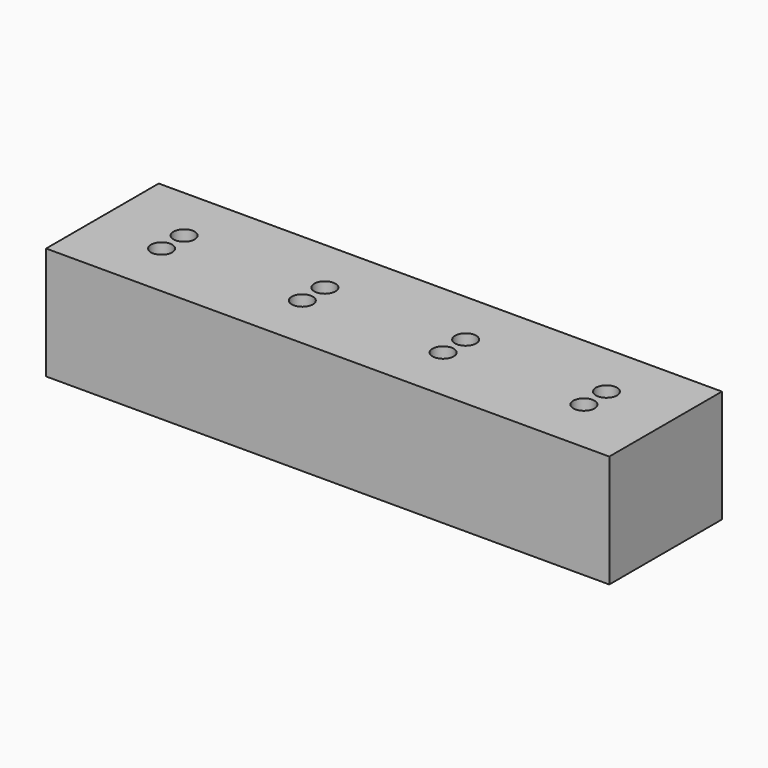
from build123d import *

# Parameters (mm, degrees)
F0_W     = 508
F0_H     = 127
F0_R     = 9.525
F1_DEPTH = 25.4
F3_DEPTH = 101.6


# Not quite as in the source:
# - a fillet or chamfer that OpenCascade refuses, or shapes differently, is made with other operations: its cross-section is extruded or revolved along the edge and cut away or added


with BuildPart() as f1:
    # F0 (on Top) → F1 (new body)
    with BuildSketch(Plane.XY):
        with Locations((254, 63.5)):
            Rectangle(F0_W, F0_H)
        with Locations((63.5, 50.8)):
            Circle(F0_R, mode=Mode.SUBTRACT)
        with Locations((190.5, 50.8)):
            Circle(F0_R, mode=Mode.SUBTRACT)
        with Locations((317.5, 50.8)):
            Circle(F0_R, mode=Mode.SUBTRACT)
        with Locations((444.5, 50.8)):
            Circle(F0_R, mode=Mode.SUBTRACT)
        with Locations((63.5, 76.2)):
            Circle(F0_R, mode=Mode.SUBTRACT)
        with Locations((190.5, 76.2)):
            Circle(F0_R, mode=Mode.SUBTRACT)
        with Locations((317.5, 76.2)):
            Circle(F0_R, mode=Mode.SUBTRACT)
        with Locations((444.5, 76.2)):
            Circle(F0_R, mode=Mode.SUBTRACT)
    extrude(amount=F1_DEPTH)

    # F2: fillet of radius 5.08 on 16 edges, made by hand

    # F2_s1 → F2_t2 (revolve, cut)
    with BuildSketch(Plane.XZ.offset(-76.2)):
        with BuildLine():
            ThreePointArc((200.025, 20.32), (201.5128975516, 23.9121024484), (205.105, 25.4))
            Line((205.105, 25.4), (200.025, 25.4))
            Line((200.025, 25.4), (200.025, 20.32))
        make_face()
    revolve(axis=Axis((190.5, 76.2, 25.4), (0, 0, 1)), mode=Mode.SUBTRACT)

    # F2_s3 → F2_t4 (revolve, cut)
    with BuildSketch(Plane.XZ.offset(-50.8)):
        with BuildLine():
            ThreePointArc((200.025, 20.32), (201.5128975516, 23.9121024484), (205.105, 25.4))
            Line((205.105, 25.4), (200.025, 25.4))
            Line((200.025, 25.4), (200.025, 20.32))
        make_face()
    revolve(axis=Axis((190.5, 50.8, 25.4), (0, 0, 1)), mode=Mode.SUBTRACT)

    # F2_s5 → F2_t6 (revolve, cut)
    with BuildSketch(Plane.XZ.offset(-76.2)):
        with BuildLine():
            ThreePointArc((327.025, 20.32), (328.5128975516, 23.9121024484), (332.105, 25.4))
            Line((332.105, 25.4), (327.025, 25.4))
            Line((327.025, 25.4), (327.025, 20.32))
        make_face()
    revolve(axis=Axis((317.5, 76.2, 25.4), (0, 0, 1)), mode=Mode.SUBTRACT)

    # F2_s7 → F2_t8 (revolve, cut)
    with BuildSketch(Plane.XZ.offset(-50.8)):
        with BuildLine():
            ThreePointArc((327.025, 20.32), (328.5128975516, 23.9121024484), (332.105, 25.4))
            Line((332.105, 25.4), (327.025, 25.4))
            Line((327.025, 25.4), (327.025, 20.32))
        make_face()
    revolve(axis=Axis((317.5, 50.8, 25.4), (0, 0, 1)), mode=Mode.SUBTRACT)

    # F2_s9 → F2_t10 (revolve, cut)
    with BuildSketch(Plane.XZ.offset(-76.2)):
        with BuildLine():
            ThreePointArc((73.025, 20.32), (74.5128975516, 23.9121024484), (78.105, 25.4))
            Line((78.105, 25.4), (73.025, 25.4))
            Line((73.025, 25.4), (73.025, 20.32))
        make_face()
    revolve(axis=Axis((63.5, 76.2, 25.4), (0, 0, 1)), mode=Mode.SUBTRACT)

    # F2_s11 → F2_t12 (revolve, cut)
    with BuildSketch(Plane.XZ.offset(-50.8)):
        with BuildLine():
            ThreePointArc((73.025, 20.32), (74.5128975516, 23.9121024484), (78.105, 25.4))
            Line((78.105, 25.4), (73.025, 25.4))
            Line((73.025, 25.4), (73.025, 20.32))
        make_face()
    revolve(axis=Axis((63.5, 50.8, 25.4), (0, 0, 1)), mode=Mode.SUBTRACT)

    # F2_s13 → F2_t14 (revolve, cut)
    with BuildSketch(Plane.XZ.offset(-76.2)):
        with BuildLine():
            ThreePointArc((454.025, 20.32), (455.5128975516, 23.9121024484), (459.105, 25.4))
            Line((459.105, 25.4), (454.025, 25.4))
            Line((454.025, 25.4), (454.025, 20.32))
        make_face()
    revolve(axis=Axis((444.5, 76.2, 25.4), (0, 0, 1)), mode=Mode.SUBTRACT)

    # F2_s15 → F2_t16 (revolve, cut)
    with BuildSketch(Plane.XZ.offset(-50.8)):
        with BuildLine():
            ThreePointArc((454.025, 20.32), (455.5128975516, 23.9121024484), (459.105, 25.4))
            Line((459.105, 25.4), (454.025, 25.4))
            Line((454.025, 25.4), (454.025, 20.32))
        make_face()
    revolve(axis=Axis((444.5, 50.8, 25.4), (0, 0, 1)), mode=Mode.SUBTRACT)

    # F2_s17 → F2_t18 (revolve, cut)
    with BuildSketch(Plane.XZ.offset(-50.8)):
        with BuildLine():
            ThreePointArc((200.025, 5.08), (201.5128975516, 1.4878975516), (205.105, 0))
            Line((205.105, 0), (200.025, 0))
            Line((200.025, 0), (200.025, 5.08))
        make_face()
    revolve(axis=Axis((190.5, 50.8, 0), (0, 0, 1)), mode=Mode.SUBTRACT)

    # F2_s19 → F2_t20 (revolve, cut)
    with BuildSketch(Plane.XZ.offset(-76.2)):
        with BuildLine():
            ThreePointArc((200.025, 5.08), (201.5128975516, 1.4878975516), (205.105, 0))
            Line((205.105, 0), (200.025, 0))
            Line((200.025, 0), (200.025, 5.08))
        make_face()
    revolve(axis=Axis((190.5, 76.2, 0), (0, 0, 1)), mode=Mode.SUBTRACT)

    # F2_s21 → F2_t22 (revolve, cut)
    with BuildSketch(Plane.XZ.offset(-50.8)):
        with BuildLine():
            ThreePointArc((327.025, 5.08), (328.5128975516, 1.4878975516), (332.105, 0))
            Line((332.105, 0), (327.025, 0))
            Line((327.025, 0), (327.025, 5.08))
        make_face()
    revolve(axis=Axis((317.5, 50.8, 0), (0, 0, 1)), mode=Mode.SUBTRACT)

    # F2_s23 → F2_t24 (revolve, cut)
    with BuildSketch(Plane.XZ.offset(-76.2)):
        with BuildLine():
            ThreePointArc((327.025, 5.08), (328.5128975516, 1.4878975516), (332.105, 0))
            Line((332.105, 0), (327.025, 0))
            Line((327.025, 0), (327.025, 5.08))
        make_face()
    revolve(axis=Axis((317.5, 76.2, 0), (0, 0, 1)), mode=Mode.SUBTRACT)

    # F2_s25 → F2_t26 (revolve, cut)
    with BuildSketch(Plane.XZ.offset(-50.8)):
        with BuildLine():
            ThreePointArc((454.025, 5.08), (455.5128975516, 1.4878975516), (459.105, 0))
            Line((459.105, 0), (454.025, 0))
            Line((454.025, 0), (454.025, 5.08))
        make_face()
    revolve(axis=Axis((444.5, 50.8, 0), (0, 0, 1)), mode=Mode.SUBTRACT)

    # F2_s27 → F2_t28 (revolve, cut)
    with BuildSketch(Plane.XZ.offset(-76.2)):
        with BuildLine():
            ThreePointArc((454.025, 5.08), (455.5128975516, 1.4878975516), (459.105, 0))
            Line((459.105, 0), (454.025, 0))
            Line((454.025, 0), (454.025, 5.08))
        make_face()
    revolve(axis=Axis((444.5, 76.2, 0), (0, 0, 1)), mode=Mode.SUBTRACT)

    # F2_s29 → F2_t30 (revolve, cut)
    with BuildSketch(Plane.XZ.offset(-76.2)):
        with BuildLine():
            ThreePointArc((73.025, 5.08), (74.5128975516, 1.4878975516), (78.105, 0))
            Line((78.105, 0), (73.025, 0))
            Line((73.025, 0), (73.025, 5.08))
        make_face()
    revolve(axis=Axis((63.5, 76.2, 0), (0, 0, 1)), mode=Mode.SUBTRACT)

    # F2_s31 → F2_t32 (revolve, cut)
    with BuildSketch(Plane.XZ.offset(-50.8)):
        with BuildLine():
            ThreePointArc((73.025, 5.08), (74.5128975516, 1.4878975516), (78.105, 0))
            Line((78.105, 0), (73.025, 0))
            Line((73.025, 0), (73.025, 5.08))
        make_face()
    revolve(axis=Axis((63.5, 50.8, 0), (0, 0, 1)), mode=Mode.SUBTRACT)

    # F0 (on Top) → F3 (join)
    with BuildSketch(Plane.XY):
        with Locations((254, 63.5)):
            Rectangle(F0_W, F0_H)
        with Locations((63.5, 50.8)):
            Circle(F0_R, mode=Mode.SUBTRACT)
        with Locations((190.5, 50.8)):
            Circle(F0_R, mode=Mode.SUBTRACT)
        with Locations((317.5, 50.8)):
            Circle(F0_R, mode=Mode.SUBTRACT)
        with Locations((444.5, 50.8)):
            Circle(F0_R, mode=Mode.SUBTRACT)
        with Locations((63.5, 76.2)):
            Circle(F0_R, mode=Mode.SUBTRACT)
        with Locations((190.5, 76.2)):
            Circle(F0_R, mode=Mode.SUBTRACT)
        with Locations((317.5, 76.2)):
            Circle(F0_R, mode=Mode.SUBTRACT)
        with Locations((444.5, 76.2)):
            Circle(F0_R, mode=Mode.SUBTRACT)
    extrude(amount=F3_DEPTH)


solid = f1.part
